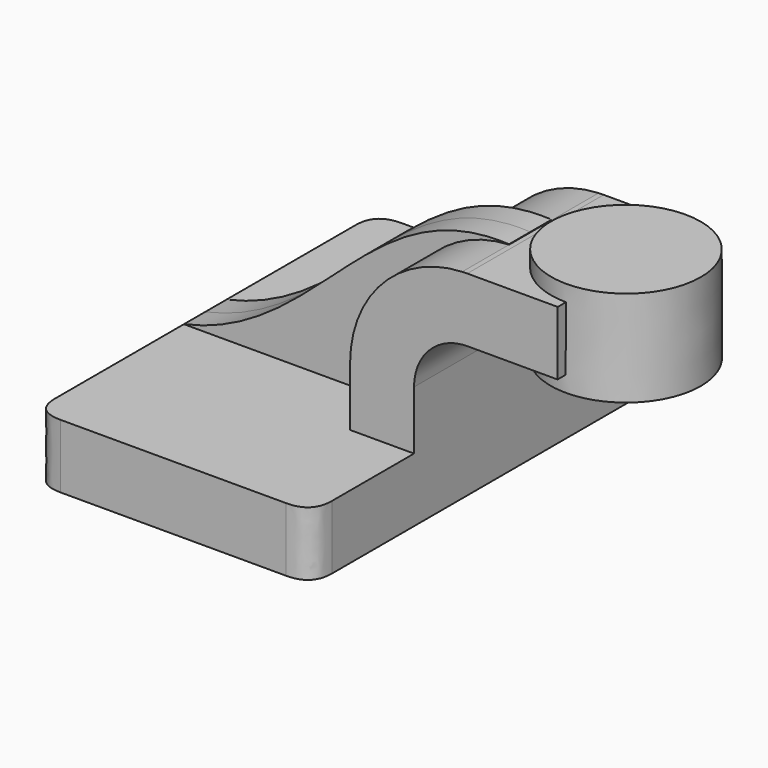
from build123d import *

# Parameters (mm, degrees)
F1_DEPTH    = 63.5
F2_DEPTH    = 25.4
F3_DEPTH    = 7.9375
F5_T1_DEPTH = 57.15


# Not quite as in the source:
# - a fillet or chamfer that OpenCascade refuses, or shapes differently, is made with other operations: its cross-section is extruded or revolved along the edge and cut away or added


with BuildPart() as f1:
    # F0 (on Front) → F1 (new body, symmetric)
    with BuildSketch(Plane.XZ):
        Polygon((-41.275, 9.525), (-41.275, -9.525), (41.275, -9.525), (41.275, 9.525), (22.225, 9.525), align=None)
    extrude(amount=F1_DEPTH, both=True)

    # F0 (on Front) → F2 (join, symmetric)
    with BuildSketch(Plane.XZ):
        with BuildLine():
            Line((22.225, 9.525), (41.275, 9.525))
            Line((41.275, 9.525), (41.275, 27.0002))
            ThreePointArc((41.275, 27.0002), (45.4000764986, 37.6751671059), (55.631525696, 42.8024106298))
            Line((55.631525696, 42.8024106298), (55.631525696, 61.8921741601))
            ThreePointArc((55.631525696, 61.8921741601), (31.9231458554, 51.1530767431), (22.225, 27.0002))
            Line((22.225, 27.0002), (22.225, 9.525))
        make_face()
        with BuildLine():
            ThreePointArc((57.15, 61.9252), (56.3905832965, 61.9169425639), (55.631525696, 61.8921741601))
            Line((55.631525696, 61.8921741601), (55.631525696, 42.8024106298))
            ThreePointArc((55.631525696, 42.8024106298), (56.3898910433, 42.8569922158), (57.15, 42.8752))
            Line((57.15, 42.8752), (84.0459217609, 42.8752))
            Line((84.0459217609, 42.8752), (84.1045851677, 61.9252))
            Line((84.1045851677, 61.9252), (57.15, 61.9252))
        make_face()
    extrude(amount=F2_DEPTH, both=True)

    # F0 (on Front) → F3 (join, symmetric)
    with BuildSketch(Plane.XZ):
        with BuildLine():
            add(Edge.make_bspline(
                [(-41.275, 9.525), (-0.4847672351, 18.3894253248), (13.3813129593, 64.201731175), (55.631525696, 62.0233434816)],
                knots=[0, 0, 0, 0, 110.1949360256, 110.1949360256, 110.1949360256, 110.1949360256], degree=3))
            Line((-41.275, 9.525), (22.225, 9.525))
            Line((22.225, 9.525), (22.225, 27.0002))
            ThreePointArc((22.225, 27.0002), (31.9231458554, 51.1530767431), (55.631525696, 61.8921741601))
            Line((55.631525696, 61.8921741601), (55.631525696, 62.0233434816))
        make_face()
    extrude(amount=F3_DEPTH, both=True)

    # F0 (on Front) → F4 (revolve)
    with BuildSketch(Plane.XZ):
        Polygon((106.431525696, 66.675), (84.1192119104, 66.675), (84.1045851677, 61.9252), (84.0459217609, 42.8752), (84.0312168002, 38.1), (106.431525696, 38.1), align=None)
    revolve(axis=Axis((84.0752143553, 0, 52.3875), (0.0030794293, 0, 0.9999952585)))

    # F5: fillet of radius 7.62 on 4 edges, made by hand

    # F5_s2 → F5_t1 (cut)
    with BuildSketch(Plane.XY.offset(-28.575)):
        with BuildLine():
            add(Edge.make_bspline(
                [(-41.275, -55.88), (-41.275, -63.5), (-33.655, -63.5)],
                knots=[0, 0, 0, 1, 1, 1], degree=2, weights=[1, 1, 1]))
            Line((-33.655, -63.5), (-41.275, -63.5))
            Line((-41.275, -63.5), (-41.275, -55.88))
        make_face()
        with BuildLine():
            add(Edge.make_bspline(
                [(33.655, -63.5), (41.275, -63.5), (41.275, -55.88)],
                knots=[0, 0, 0, 1, 1, 1], degree=2, weights=[1, 1, 1]))
            Line((41.275, -55.88), (41.275, -63.5))
            Line((41.275, -63.5), (33.655, -63.5))
        make_face()
        with BuildLine():
            add(Edge.make_bspline(
                [(-41.275, 55.88), (-41.275, 63.5), (-33.655, 63.5)],
                knots=[0, 0, 0, 1, 1, 1], degree=2, weights=[1, 1, 1]))
            Line((-33.655, 63.5), (-41.275, 63.5))
            Line((-41.275, 63.5), (-41.275, 55.88))
        make_face()
        with BuildLine():
            add(Edge.make_bspline(
                [(33.655, 63.5), (41.275, 63.5), (41.275, 55.88)],
                knots=[0, 0, 0, 1, 1, 1], degree=2, weights=[1, 1, 1]))
            Line((41.275, 55.88), (41.275, 63.5))
            Line((41.275, 63.5), (33.655, 63.5))
        make_face()
    extrude(amount=F5_T1_DEPTH, mode=Mode.SUBTRACT)


solid = f1.part
